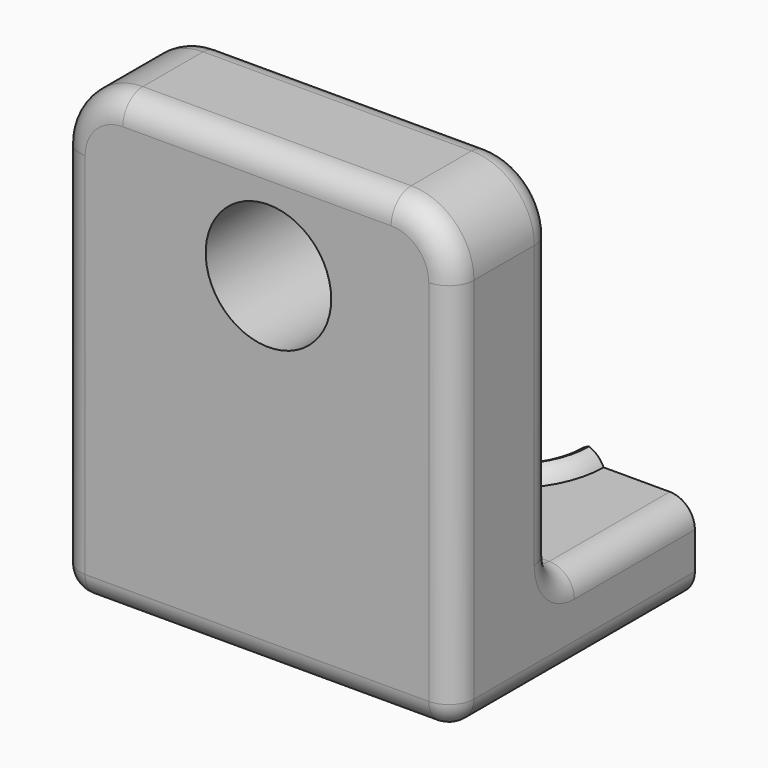
from build123d import *

# Parameters (mm, degrees)
F0_W         = 79.6983499915
F0_H         = 74.7635825602
F0_R         = 12.7
F0_H_2       = 17.6352638877
F1_DEPTH     = 25.4
F2_DEPTH     = 35.56
F4_DEPTH     = 17.6362638877
F5_R         = 12.7
F6_R         = 5.08
F7_T1_DEPTH  = 69.5383499915
F7_S5_W      = 5.08
F7_S5_H      = 5.08
F7_T6_DEPTH  = 5.08
F7_S11_W     = 5.08
F7_S11_H     = 5.08
F7_T12_DEPTH = 5.08
F8_DEPTH     = 3.048
F9_T2_ANGLE  = 250.1291990291
F9_T4_ANGLE  = 294.7758439205


# Not quite as in the source:
# - a fillet or chamfer that OpenCascade refuses, or shapes differently, is made with other operations: its cross-section is extruded or revolved along the edge and cut away or added


with BuildPart() as f1:
    # F0 (on Front) → F1 (new body)
    with BuildSketch(Plane.XZ):
        with Locations((-2.3253131658, 16.0799051921)):
            Rectangle(F0_W, F0_H)
        with Locations((0, 31.3866536387)):
            Circle(F0_R, mode=Mode.SUBTRACT)
        with Locations((-2.3253131658, -30.1195180319)):
            Rectangle(F0_W, F0_H_2)
    extrude(amount=F1_DEPTH)

    # F0 (on Front) → F2 (join)
    with BuildSketch(Plane.XZ):
        with Locations((-2.3253131658, -30.1195180319)):
            Rectangle(F0_W, F0_H_2)
    extrude(amount=-F2_DEPTH)

    # F3 (on face) → F4 (cut, through all)
    with BuildSketch(Plane.XY.offset(-21.3018860881)):
        with BuildLine():
            ThreePointArc((-12.7, 35.56), (0, 22.86), (12.7, 35.56))
            Line((12.7, 35.56), (-12.7, 35.56))
        make_face()
    extrude(amount=-F4_DEPTH, mode=Mode.SUBTRACT)

    # F5
    f5_edges = [f1.edges().sort_by_distance(p)[0] for p in [
        (-42.174488, -12.7, 53.461696),
        (37.523862, -12.7, 53.461696),
    ]]
    fillet(f5_edges, radius=F5_R)

    # F6
    f6_edges = [f1.edges().sort_by_distance(p)[0] for p in [
        (-2.325313, 0, 53.461696),
        (-2.325313, -25.4, 53.461696),
        (-42.174488, 0, 9.729905),
        (37.523862, 0, 9.729905),
        (-2.325313, 0, -21.301886),
        (37.523862, 17.78, -21.301886),
        (-42.174488, 17.78, -21.301886),
        (-42.174488, -25.4, 0.912273),
        (-42.174488, 5.08, -38.93715),
        (37.523862, -25.4, 0.912273),
        (37.523862, 5.08, -38.93715),
    ]]
    fillet(f6_edges, radius=F6_R)

    # F7: fillet of radius 5.08 on 1 edges, made by hand

    # F7_s2 → F7_t1 (cut)
    with BuildSketch(Plane.YZ.offset(-37.0944881615)):
        with BuildLine():
            ThreePointArc((-25.4, -33.8571499758), (-23.9121024484, -37.4492524242), (-20.32, -38.9371499758))
            Line((-20.32, -38.9371499758), (-25.4, -38.9371499758))
            Line((-25.4, -38.9371499758), (-25.4, -33.8571499758))
        make_face()
    extrude(amount=F7_T1_DEPTH, mode=Mode.SUBTRACT)


with BuildPart() as f7_tool4:
    # F7_s5 → F7_t6 (new body)
    with BuildSketch(Plane.XZ.offset(20.32)):
        with Locations((-39.6344881615, -36.3971499758)):
            Rectangle(F7_S5_W, F7_S5_H)
    extrude(amount=F7_T6_DEPTH)

    # F7_s7 → F7_t8 (revolve, cut)
    with BuildSketch(Plane(origin=(-37.0944881615, -20.32, -33.8571499758), x_dir=(0.7071067812, 0, 0.7071067812), z_dir=(0.7071067812, 0, -0.7071067812))):
        with BuildLine():
            ThreePointArc((0, -5.08), (5.08, 0), (0, 5.08))
            Line((0, 5.08), (0, -5.08))
        make_face()
    revolve(axis=Axis((-37.0944881615, -20.32, -33.8571499758), (0, -1, 0)), mode=Mode.SUBTRACT)


with BuildPart() as f1_1:
    add(f1.part)

    # F7_t3: cut F7_tool4
    add(f7_tool4.part, mode=Mode.SUBTRACT)


with BuildPart() as f7_tool10:
    # F7_s11 → F7_t12 (new body)
    with BuildSketch(Plane.XZ.offset(20.32)):
        with Locations((34.98386183, -36.3971499758)):
            Rectangle(F7_S11_W, F7_S11_H)
    extrude(amount=F7_T12_DEPTH)

    # F7_s13 → F7_t14 (revolve, cut)
    with BuildSketch(Plane(origin=(32.44386183, -20.32, -33.8571499758), x_dir=(-0.7071067812, 0, 0.7071067812), z_dir=(0.7071067812, 0, 0.7071067812))):
        with BuildLine():
            ThreePointArc((0, -5.08), (5.08, 0), (0, 5.08))
            Line((0, 5.08), (0, -5.08))
        make_face()
    revolve(axis=Axis((32.44386183, -20.32, -33.8571499758), (0, -1, 0)), mode=Mode.SUBTRACT)


with BuildPart() as f1_2:
    add(f1_1.part)

    # F7_t9: cut F7_tool10
    add(f7_tool10.part, mode=Mode.SUBTRACT)

    # F3 (on face) → F8 (join)
    with BuildSketch(Plane.XY.offset(-21.3018860881)):
        with BuildLine():
            Line((19.05, 35.56), (12.7, 35.56))
            ThreePointArc((12.7, 35.56), (0, 22.86), (-12.7, 35.56))
            Line((-12.7, 35.56), (-19.05, 35.56))
            ThreePointArc((-19.05, 35.56), (0, 16.51), (19.05, 35.56))
        make_face()
    extrude(amount=F8_DEPTH)

    # F9: fillet of radius 5.08 on 2 edges, made by hand

    # F9_s1 → F9_t2 (revolve, cut)
    with BuildSketch(Plane(origin=(16.7214049162, 23.823427639, 0), x_dir=(0, 0, 1), z_dir=(0.5744996444, 0.8185048311, 0))):
        with BuildLine():
            ThreePointArc((-21.3018860881, -39.4792073551), (-19.0836531533, -37.6057410411), (-18.2538860881, -34.823310449))
            Line((-18.2538860881, -34.823310449), (-18.2538860881, -39.4792073551))
            Line((-18.2538860881, -39.4792073551), (-21.3018860881, -39.4792073551))
        make_face()
    revolve(axis=Axis((0, 35.56, -18.2538860881), (0, 0, 1)), revolution_arc=F9_T2_ANGLE, mode=Mode.SUBTRACT)

    # F9_s3 → F9_t4 (revolve, cut)
    with BuildSketch(Plane(origin=(-16.14342639, 10.3289474307, 0), x_dir=(0, 0, 1), z_dir=(-0.8423388046, 0.5389483633, 0))):
        with BuildLine():
            ThreePointArc((-18.2538860881, 47.7335678904), (-19.7417836396, 44.141465442), (-23.3338860881, 42.6535678904))
            Line((-23.3338860881, 42.6535678904), (-18.2538860881, 42.6535678904))
            Line((-18.2538860881, 42.6535678904), (-18.2538860881, 47.7335678904))
        make_face()
    revolve(axis=Axis((0, 35.56, -18.2538860881), (0, 0, -1)), revolution_arc=F9_T4_ANGLE, mode=Mode.SUBTRACT)


solid = f1_2.part
